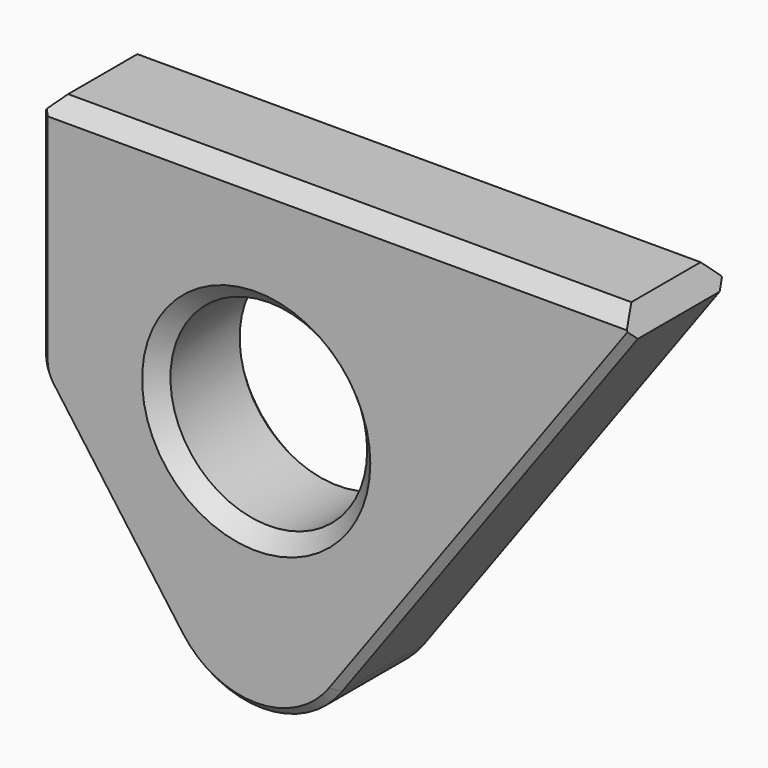
from build123d import *

# Parameters (mm, degrees)
F1_DEPTH    = 15
F2_T1_DEPTH = 34.8219363514
F2_T3_DEPTH = 25.2867319519
F2_T5_DEPTH = 87.7867319519
F3_R        = 5
F4_SIZE     = 1


# Not quite as in the source:
# - a fillet or chamfer that OpenCascade refuses, or shapes differently, is made with other operations: its cross-section is extruded or revolved along the edge and cut away or added


with BuildPart() as f1:
    # F0 (on Front) → F1 (new body)
    with BuildSketch(Plane.XZ):
        with BuildLine():
            Line((50, 60), (0, 60))
            Line((0, 60), (-27.5, 60))
            Line((-27.5, 60), (-27.5, 29.0612040202))
            Line((-27.5, 29.0612040202), (-10.1093475479, 5.1480552127))
            ThreePointArc((-10.1093475479, 5.1480552127), (0, 0), (10.1093475479, 5.1480552127))
            Line((10.1093475479, 5.1480552127), (50, 60))
        make_face()
        with BuildLine():
            ThreePointArc((12.5, 32.5), (-8.8388347648, 23.6611652352), (0, 45))
            ThreePointArc((0, 45), (8.8388347648, 41.3388347648), (12.5, 32.5))
        make_face(mode=Mode.SUBTRACT)
    extrude(amount=F1_DEPTH)

    # F2: chamfer of 2 on 7 edges, made by hand

    # F2_s2 → F2_t1 (cut)
    with BuildSketch(Plane.XZ.offset(-9.9109681757)):
        Polygon((47.69005228, 56.823688834), (46.0725566723, 60), (50, 60), align=None)
    extrude(amount=F2_T1_DEPTH, mode=Mode.SUBTRACT)

    # F2_s4 → F2_t3 (cut)
    with BuildSketch(Plane.XZ.offset(-5.1433659759)):
        Polygon((-25.5, 60), (-27.5, 58), (-27.5, 60), align=None)
    extrude(amount=F2_T3_DEPTH, mode=Mode.SUBTRACT)

    # F2_s6 → F2_t5 (cut)
    with BuildSketch(Plane.YZ.offset(-32.6433659759)):
        Polygon((-2, 60), (0, 58), (0, 60), align=None)
        Polygon((-13, 60), (-15, 58), (-15, 60), align=None)
    extrude(amount=F2_T5_DEPTH, mode=Mode.SUBTRACT)

    # F2_s7 → F2_t8 (revolve, cut)
    with BuildSketch(Plane.XY.offset(32.5)):
        Polygon((12.5, -2), (14.5, 0), (12.5, 0), align=None)
    revolve(axis=Axis((0, 0, 32.5), (0, 1, 0)), mode=Mode.SUBTRACT)

    # F2_s9 → F2_t10 (revolve, cut)
    with BuildSketch(Plane.XY.offset(32.5)):
        Polygon((12.5, -13), (14.5, -15), (12.5, -15), align=None)
    revolve(axis=Axis((0, -15, 32.5), (0, 1, 0)), mode=Mode.SUBTRACT)

    # F3
    f3_edges = [f1.edges().sort_by_distance(p)[0] for p in [
        (-27.5, -7.5, 29.061204),
    ]]
    fillet(f3_edges, radius=F3_R)

    # F4
    f4_edges = [f1.edges().sort_by_distance(p)[0] for p in [
        (28.8997, -15, 30.985872),
        (28.8997, 0, 30.985872),
        (-27.5, 0, 44.343534),
        (-27.254929, 0, 29.140895),
        (-18.326543, 0, 16.447173),
        (0, 0, 0),
        (-27.5, -15, 44.343534),
        (-27.254929, -15, 29.140895),
        (-18.326543, -15, 16.447173),
        (0, -15, 0),
    ]]
    chamfer(f4_edges, length=F4_SIZE)


solid = f1.part
